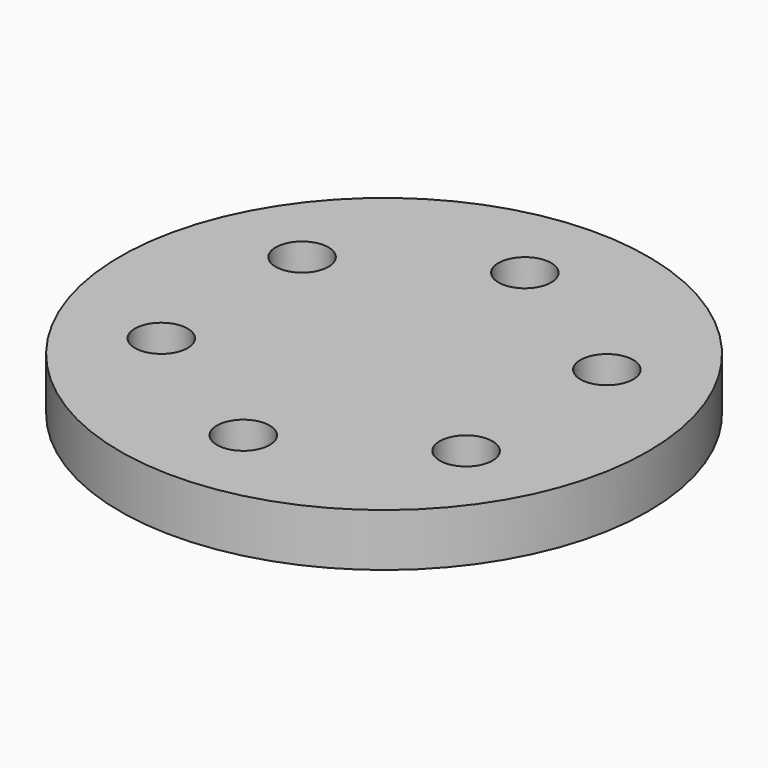
from build123d import *

# Parameters (mm, degrees)
F2_R            = 60
F3_DEPTH        = 12
F4_R            = 6
F5_DEPTH        = 12.001
F5_COPIES_COUNT = 6


# Not quite as in the source:
# - a pattern or mirror of a feature is missing from the dataset's text; its kind, count and spacing are read off the source's solid


with BuildPart() as f3:
    # F2 (on Top) → F3 (new body)
    with BuildSketch(Plane.XY):
        Circle(F2_R)
    extrude(amount=-F3_DEPTH)

    # F4 (on face) → F5 (cut, through all)
    with BuildSketch(Plane.XY):
        with Locations((0, 40)):
            Circle(F4_R)
    f5 = extrude(amount=-F5_DEPTH, mode=Mode.SUBTRACT)

    # F5_copies: F5 ×6 about axis
    f5_copies_axis = Axis((0, 0, 0), (0, 0, 1))
    for i in range(1, F5_COPIES_COUNT):
        add(f5.rotate(f5_copies_axis, i * 360 / F5_COPIES_COUNT), mode=Mode.SUBTRACT)


solid = f3.part
